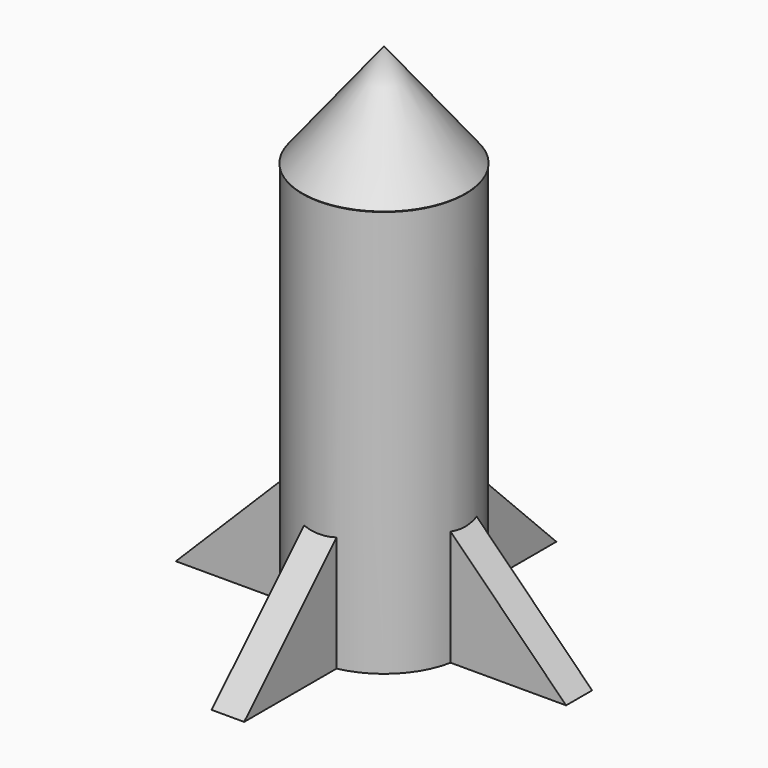
from build123d import *

# Parameters (mm, degrees)
F0_R            = 25
F1_DEPTH        = 125
F3_DEPTH        = 5
F3_COPIES_COUNT = 4


# Not quite as in the source:
# - a pattern or mirror of a feature is missing from the dataset's text; its kind, count and spacing are read off the source's solid


with BuildPart() as f1:
    # F0 (on Top) → F1 (new body)
    with BuildSketch(Plane.XY):
        Circle(F0_R)
    extrude(amount=F1_DEPTH)

    # F2 (on Front) → F3 (join, symmetric)
    with BuildSketch(Plane.XZ):
        Polygon((0, 60), (0, 0), (60, 0), align=None)
    f3 = extrude(amount=F3_DEPTH, both=True)

    # F3_copies: F3 ×4 about axis
    f3_copies_axis = Axis((0, 0, 0), (0, 0, 1))
    for i in range(1, F3_COPIES_COUNT):
        add(f3.rotate(f3_copies_axis, i * 360 / F3_COPIES_COUNT))

    # F4 (on Front) → F5 (revolve)
    with BuildSketch(Plane.XZ):
        Polygon((0, 156.9369882345), (-25.1428224146, 125.2296715975), (0, 124.8316764832), align=None)
    revolve(axis=Axis((0, 0, 140.8843323588), (0, 0, -1)))


solid = f1.part
